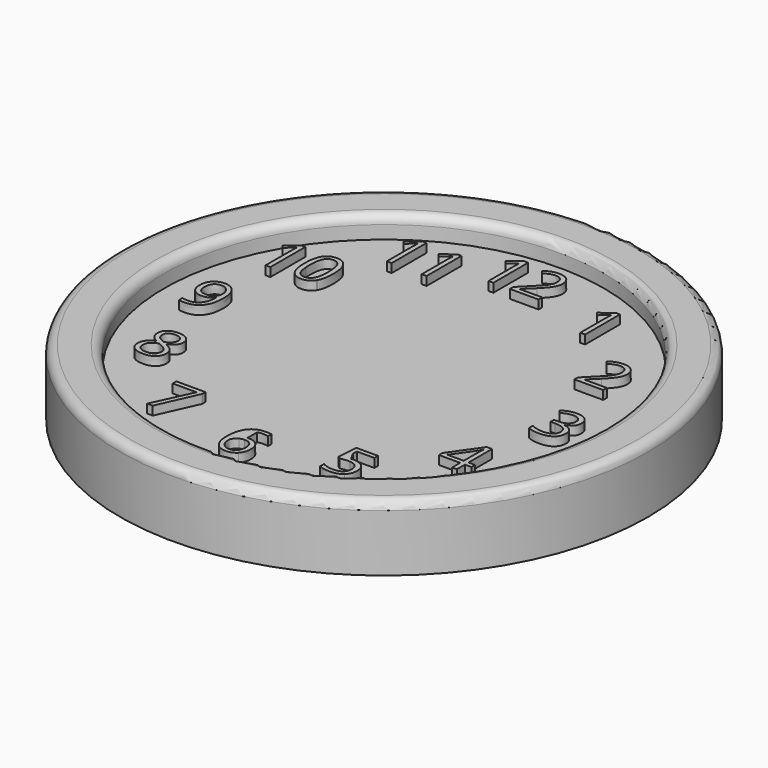
from build123d import *

# Parameters (mm, degrees)
F0_R         = 127
F1_DEPTH     = 25.4
F0_R_2       = 152.4
F2_DEPTH     = 38.1
F3_R         = 5.08
F5_TEXT_SIZE = 35.2777777778
F6_DEPTH     = 5.08


# Not quite as in the source:
# - Text() gives the source's letters only with a copy of the font that has no kerning and outlines rounded to 1/6400 em; it was checked with that copy


with BuildPart() as f1:
    # F0 (on Top) → F1 (new body)
    with BuildSketch(Plane.XY):
        Circle(F0_R)
    extrude(amount=F1_DEPTH)


with BuildPart() as f2:
    # F0 (on Top) → F2 (new body)
    with BuildSketch(Plane.XY):
        Circle(F0_R_2)
        Circle(F0_R, mode=Mode.SUBTRACT)
    extrude(amount=F2_DEPTH)

    # F3
    f3_edges = [f2.edges().sort_by_distance(p)[0] for p in [
        (-127, 0, 38.1),
        (-152.4, 0, 38.1),
    ]]
    fillet(f3_edges, radius=F3_R)


with BuildPart() as f6:
    # F5 (on offset) → F6 (new body)
    with BuildSketch(Plane.XY.offset(25.654)):
        with BuildLine():
            add(Edge.make_bspline(
                [(0, -89.0715853715), (1.4167514722, -88.7566840278), (3.0702690972, -88.7566840278)],
                knots=[0.7073397651, 0.7073397651, 0.7073397651, 1, 1, 1], degree=2))
            Line((0, -89.0715853715), (0, -91.5732459323))
            add(Edge.make_bspline(
                [(3.1033420139, -91.1158854167), (1.3779739805, -91.1158854167), (0, -91.5732459323)],
                knots=[0, 0, 0, 0.4258661898, 0.4258661898, 0.4258661898], degree=2))
            add(Edge.make_bspline(
                [(6.1350260417, -91.5458333333), (4.8065972222, -91.1158854167), (3.1033420139, -91.1158854167)],
                knots=[0, 0, 0, 1, 1, 1], degree=2))
            Line((6.1350260417, -91.5458333333), (6.1350260417, -89.0819010417))
            add(Edge.make_bspline(
                [(3.0702690972, -88.7566840278), (5.0160590278, -88.7566840278), (6.1350260417, -89.0819010417)],
                knots=[0, 0, 0, 1, 1, 1], degree=2))
        make_face()
        with BuildLine():
            Line((0, -91.5732459323), (0, -89.0715853715))
            add(Edge.make_bspline(
                [(-5.4652994792, -92.4332899306), (-3.4241913797, -89.832680375), (0, -89.0715853715)],
                knots=[0, 0, 0, 0.7073397651, 0.7073397651, 0.7073397651], degree=2))
            add(Edge.make_bspline(
                [(-8.3509114583, -103.534765625), (-8.3509114583, -96.1098958333), (-5.4652994792, -92.4332899306)],
                knots=[0, 0, 0, 1, 1, 1], degree=2))
            add(Edge.make_bspline(
                [(-6.0606119792, -111.7092881944), (-8.3509114583, -108.7713107639), (-8.3509114583, -103.534765625)],
                knots=[0, 0, 0, 1, 1, 1], degree=2))
            add(Edge.make_bspline(
                [(0.1378038194, -114.647265625), (-3.7703125, -114.647265625), (-6.0606119792, -111.7092881944)],
                knots=[0, 0, 0, 1, 1, 1], degree=2))
            add(Edge.make_bspline(
                [(5.9365885417, -112.3983072917), (3.7923611111, -114.647265625), (0.1378038194, -114.647265625)],
                knots=[0, 0, 0, 1, 1, 1], degree=2))
            add(Edge.make_bspline(
                [(8.0808159722, -106.2191840278), (8.0808159722, -110.1493489583), (5.9365885417, -112.3983072917)],
                knots=[0, 0, 0, 1, 1, 1], degree=2))
            add(Edge.make_bspline(
                [(6.1267578125, -100.657421875), (8.0808159722, -102.7079427083), (8.0808159722, -106.2191840278)],
                knots=[0, 0, 0, 1, 1, 1], degree=2))
            add(Edge.make_bspline(
                [(0.7772135417, -98.6069010417), (4.1726996528, -98.6069010417), (6.1267578125, -100.657421875)],
                knots=[0, 0, 0, 1, 1, 1], degree=2))
            add(Edge.make_bspline(
                [(0, -98.6349784999), (0.378169054, -98.6069010417), (0.7772135417, -98.6069010417)],
                knots=[0.9026967975, 0.9026967975, 0.9026967975, 1, 1, 1], degree=2))
            add(Edge.make_bspline(
                [(-5.2200086806, -101.5724392361), (-3.5083325655, -98.8954574051), (0, -98.6349784999)],
                knots=[0, 0, 0, 0.9026967975, 0.9026967975, 0.9026967975], degree=2))
            Line((-5.2200086806, -101.5724392361), (-5.4239583333, -101.5724392361))
            add(Edge.make_bspline(
                [(-3.0840494792, -93.6376953125), (-5.2200086806, -96.1595052083), (-5.4239583333, -101.5724392361)],
                knots=[0, 0, 0, 1, 1, 1], degree=2))
            add(Edge.make_bspline(
                [(0, -91.5732459323), (-1.8577230845, -92.1898389885), (-3.0840494792, -93.6376953125)],
                knots=[0.4258661898, 0.4258661898, 0.4258661898, 1, 1, 1], degree=2))
        make_face()
        with BuildLine():
            add(Edge.make_bspline(
                [(0, -100.8653424744), (-1.4082443896, -100.9117606324), (-2.5989800347, -101.50078125)],
                knots=[0.0788056591, 0.0788056591, 0.0788056591, 1, 1, 1], degree=2))
            add(Edge.make_bspline(
                [(0.2425347222, -100.8613715278), (0.1204714602, -100.8613715278), (0, -100.8653424744)],
                knots=[0, 0, 0, 0.0788056591, 0.0788056591, 0.0788056591], degree=2))
            add(Edge.make_bspline(
                [(3.9963107639, -102.2917751736), (2.7395399306, -100.8613715278), (0.2425347222, -100.8613715278)],
                knots=[0, 0, 0, 1, 1, 1], degree=2))
            add(Edge.make_bspline(
                [(5.2530815972, -106.2191840278), (5.2530815972, -103.7221788194), (3.9963107639, -102.2917751736)],
                knots=[0, 0, 0, 1, 1, 1], degree=2))
            add(Edge.make_bspline(
                [(3.9026041667, -110.6730034722), (5.2530815972, -109.1296006944), (5.2530815972, -106.2191840278)],
                knots=[0, 0, 0, 1, 1, 1], degree=2))
            add(Edge.make_bspline(
                [(0.1047309028, -112.21640625), (2.5521267361, -112.21640625), (3.9026041667, -110.6730034722)],
                knots=[0, 0, 0, 1, 1, 1], degree=2))
            add(Edge.make_bspline(
                [(-2.7808810764, -111.3206814236), (-1.5158420139, -112.21640625), (0.1047309028, -112.21640625)],
                knots=[0, 0, 0, 1, 1, 1], degree=2))
            add(Edge.make_bspline(
                [(-4.7349392361, -108.892578125), (-4.0459201389, -110.4249565972), (-2.7808810764, -111.3206814236)],
                knots=[0, 0, 0, 1, 1, 1], degree=2))
            add(Edge.make_bspline(
                [(-5.4239583333, -105.5852864583), (-5.4239583333, -107.3601996528), (-4.7349392361, -108.892578125)],
                knots=[0, 0, 0, 1, 1, 1], degree=2))
            add(Edge.make_bspline(
                [(-4.6577690972, -103.2591579861), (-5.4239583333, -104.378125), (-5.4239583333, -105.5852864583)],
                knots=[0, 0, 0, 1, 1, 1], degree=2))
            add(Edge.make_bspline(
                [(-2.5989800347, -101.50078125), (-3.8915798611, -102.1401909722), (-4.6577690972, -103.2591579861)],
                knots=[0, 0, 0, 1, 1, 1], degree=2))
        make_face(mode=Mode.SUBTRACT)
        Polygon((44.4279513889, -75.5031549828), (44.3256858106, -76.7743399042), (46.6502291754, -80.8005671165), (46.8753472222, -78.1379640106), (56.9515625, -78.1379640106), (56.9515625, -75.5031549828), align=None)
        with BuildLine():
            Line((46.6502291754, -80.8005671165), (44.3256858106, -76.7743399042))
            Line((44.3256858106, -76.7743399042), (43.4798611111, -87.2881376217))
            Line((43.4798611111, -87.2881376217), (44.9626302083, -88.2362278995))
            add(Edge.make_bspline(
                [(49.3392795139, -87.7346219967), (47.7021701389, -87.7346219967), (44.9626302083, -88.2362278995)],
                knots=[0, 0, 0, 1, 1, 1], degree=2))
            add(Edge.make_bspline(
                [(50.690992768, -87.7993749604), (50.0547939445, -87.7346219967), (49.3392795139, -87.7346219967)],
                knots=[0.8891488365, 0.8891488365, 0.8891488365, 1, 1, 1], degree=2))
            Line((50.690992768, -87.7993749604), (49.2626542608, -85.3254200954))
            add(Edge.make_bspline(
                [(46.2359375, -85.7006376217), (47.7525335288, -85.3964735157), (49.2626542608, -85.3254200954)],
                knots=[0, 0, 0, 0.7663977475, 0.7663977475, 0.7663977475], degree=2))
            Line((46.2359375, -85.7006376217), (46.6502291754, -80.8005671165))
        make_face()
        with BuildLine():
            add(Edge.make_bspline(
                [(-71.6590054686, 41.3723460972), (-71.7749145216, 41.167531428), (-71.8982070662, 40.9745876736)],
                knots=[0.9401140472, 0.9401140472, 0.9401140472, 1, 1, 1], degree=2))
            Line((-71.6590054686, 41.3723460972), (-74.0546251018, 42.7554577373))
            add(Edge.make_bspline(
                [(-78.1958416148, 40.2166666667), (-75.3363356992, 40.2166666667), (-74.0546251018, 42.7554577373)],
                knots=[0, 0, 0, 0.9995451018, 0.9995451018, 0.9995451018], degree=2))
            add(Edge.make_bspline(
                [(-82.3106636634, 42.7246961806), (-81.018063837, 40.2166666667), (-78.1958416148, 40.2166666667)],
                knots=[0, 0, 0, 1, 1, 1], degree=2))
            add(Edge.make_bspline(
                [(-83.5262787662, 48.2239195301), (-83.2878107352, 44.6206531855), (-82.3106636634, 42.7246961806)],
                knots=[0.2440451779, 0.2440451779, 0.2440451779, 1, 1, 1], degree=2))
            Line((-83.5262787662, 48.2239195301), (-86.4886726615, 49.934258443))
            add(Edge.make_bspline(
                [(-84.3777209551, 41.0517578125), (-86.3631522517, 44.1422145902), (-86.4886726615, 49.934258443)],
                knots=[0, 0, 0, 0.9367792731, 0.9367792731, 0.9367792731], degree=2))
            add(Edge.make_bspline(
                [(-78.1958416148, 37.752734375), (-82.258298212, 37.752734375), (-84.3777209551, 41.0517578125)],
                knots=[0, 0, 0, 1, 1, 1], degree=2))
            add(Edge.make_bspline(
                [(-71.8982070662, 40.9745876736), (-73.9569961287, 37.752734375), (-78.1958416148, 37.752734375)],
                knots=[0, 0, 0, 1, 1, 1], degree=2))
        make_face()
        with BuildLine():
            Line((-74.0546251018, 42.7554577373), (-71.6590054686, 41.3723460972))
            add(Edge.make_bspline(
                [(-69.8394180037, 50.7283420139), (-69.8394180037, 44.5876100894), (-71.6590054686, 41.3723460972)],
                knots=[0, 0, 0, 0.9401140472, 0.9401140472, 0.9401140472], degree=2))
            add(Edge.make_bspline(
                [(-71.9671089759, 60.3553168403), (-69.8394180037, 57.0287326389), (-69.8394180037, 50.7283420139)],
                knots=[0, 0, 0, 1, 1, 1], degree=2))
            add(Edge.make_bspline(
                [(-78.1958416148, 63.6819010417), (-74.0947999481, 63.6819010417), (-71.9671089759, 60.3553168403)],
                knots=[0, 0, 0, 1, 1, 1], degree=2))
            add(Edge.make_bspline(
                [(-84.4466228648, 60.4931206597), (-82.3961020314, 63.6819010417), (-78.1958416148, 63.6819010417)],
                knots=[0, 0, 0, 1, 1, 1], degree=2))
            add(Edge.make_bspline(
                [(-86.4971436981, 50.7283420139), (-86.4971436981, 57.3043402778), (-84.4466228648, 60.4931206597)],
                knots=[0, 0, 0, 1, 1, 1], degree=2))
            add(Edge.make_bspline(
                [(-86.4886726615, 49.934258443), (-86.4971436981, 50.3251479866), (-86.4971436981, 50.7283420139)],
                knots=[0.9367792731, 0.9367792731, 0.9367792731, 1, 1, 1], degree=2))
            Line((-86.4886726615, 49.934258443), (-83.5262787662, 48.2239195301))
            add(Edge.make_bspline(
                [(-83.6032634898, 50.7283420139), (-83.6032634898, 49.3871633515), (-83.5262787662, 48.2239195301)],
                knots=[0, 0, 0, 0.2440451779, 0.2440451779, 0.2440451779], degree=2))
            add(Edge.make_bspline(
                [(-82.3106636634, 58.7126953125), (-83.6032634898, 56.2239583333), (-83.6032634898, 50.7283420139)],
                knots=[0, 0, 0, 1, 1, 1], degree=2))
            add(Edge.make_bspline(
                [(-78.1958416148, 61.2014322917), (-81.018063837, 61.2014322917), (-82.3106636634, 58.7126953125)],
                knots=[0, 0, 0, 1, 1, 1], degree=2))
            add(Edge.make_bspline(
                [(-74.0534588023, 58.6768663194), (-75.3350343231, 61.2014322917), (-78.1958416148, 61.2014322917)],
                knots=[0, 0, 0, 1, 1, 1], degree=2))
            add(Edge.make_bspline(
                [(-72.7718832814, 50.7283420139), (-72.7718832814, 56.1523003472), (-74.0534588023, 58.6768663194)],
                knots=[0, 0, 0, 1, 1, 1], degree=2))
            add(Edge.make_bspline(
                [(-74.0534588023, 42.7577690972), (-72.7718832814, 45.2988715278), (-72.7718832814, 50.7283420139)],
                knots=[0, 0, 0, 1, 1, 1], degree=2))
            add(Edge.make_bspline(
                [(-74.0546251018, 42.7554577373), (-74.0540417887, 42.7566131543), (-74.0534588023, 42.7577690972)],
                knots=[0.9995451018, 0.9995451018, 0.9995451018, 1, 1, 1], degree=2))
        make_face()
        with Locations((77.1127035939, -63.5)):
            Text('4', F5_TEXT_SIZE, font='Open Sans', text_align=(TextAlign.LEFT, TextAlign.BOTTOM))
        with Locations((-111.8829210069, -12.7)):
            Text('9', F5_TEXT_SIZE, font='Open Sans', text_align=(TextAlign.LEFT, TextAlign.BOTTOM))
        with Locations((91.4052734375, -12.7)):
            Text('3', F5_TEXT_SIZE, font='Open Sans', text_align=(TextAlign.LEFT, TextAlign.BOTTOM))
        with Locations((-98.3041749481, -63.5)):
            Text('8', F5_TEXT_SIZE, font='Open Sans', text_align=(TextAlign.LEFT, TextAlign.BOTTOM))
        Polygon((-42.7550130208, -75.5031549828), (-43.591766854, -75.5031549828), (-48.5063558794, -84.0154728732), (-56.2212022569, -100.6881810245), (-53.0517144097, -100.6881810245), (-42.7550130208, -77.7962105384), align=None)
        Polygon((-48.5063558794, -84.0154728732), (-43.591766854, -75.5031549828), (-59.5119574653, -75.5031549828), (-59.5119574653, -78.1379640106), (-45.7866970486, -78.1379640106), align=None)
        with BuildLine():
            Line((0, -98.6349784999), (0, -91.5732459323))
            add(Edge.make_bspline(
                [(0, -91.5732459323), (-1.8577230845, -92.1898389885), (-3.0840494792, -93.6376953125)],
                knots=[0.4258661898, 0.4258661898, 0.4258661898, 1, 1, 1], degree=2))
            add(Edge.make_bspline(
                [(-3.0840494792, -93.6376953125), (-5.2200086806, -96.1595052083), (-5.4239583333, -101.5724392361)],
                knots=[0, 0, 0, 1, 1, 1], degree=2))
            Line((-5.4239583333, -101.5724392361), (-5.2200086806, -101.5724392361))
            add(Edge.make_bspline(
                [(-5.2200086806, -101.5724392361), (-3.5083325655, -98.8954574051), (0, -98.6349784999)],
                knots=[0, 0, 0, 0.9026967975, 0.9026967975, 0.9026967975], degree=2))
        make_face()
        with BuildLine():
            Line((49.2626542608, -85.3254200954), (46.6502291754, -80.8005671165))
            Line((46.6502291754, -80.8005671165), (46.2359375, -85.7006376217))
            add(Edge.make_bspline(
                [(46.2359375, -85.7006376217), (47.7525335288, -85.3964735157), (49.2626542608, -85.3254200954)],
                knots=[0, 0, 0, 0.7663977475, 0.7663977475, 0.7663977475], degree=2))
        make_face()
        with BuildLine():
            add(Edge.make_bspline(
                [(49.2626542608, -85.3254200954), (49.7229473731, -85.3037626217), (50.1826388889, -85.3037626217)],
                knots=[0.7663977475, 0.7663977475, 0.7663977475, 1, 1, 1], degree=2))
            Line((49.2626542608, -85.3254200954), (50.690992768, -87.7993749604))
            add(Edge.make_bspline(
                [(55.7940104167, -93.0042400523), (55.7940104167, -88.3187652894), (50.690992768, -87.7993749604)],
                knots=[0, 0, 0, 0.8891488365, 0.8891488365, 0.8891488365], degree=2))
            add(Edge.make_bspline(
                [(54.1155598958, -97.141110712), (55.7940104167, -95.7107070662), (55.7940104167, -93.0042400523)],
                knots=[0, 0, 0, 1, 1, 1], degree=2))
            add(Edge.make_bspline(
                [(49.4054253472, -98.5715143578), (52.437109375, -98.5715143578), (54.1155598958, -97.141110712)],
                knots=[0, 0, 0, 1, 1, 1], degree=2))
            add(Edge.make_bspline(
                [(45.8721354167, -98.1305421356), (47.6635850694, -98.5715143578), (49.4054253472, -98.5715143578)],
                knots=[0, 0, 0, 1, 1, 1], degree=2))
            add(Edge.make_bspline(
                [(42.8790364583, -96.9178685245), (44.0806857639, -97.6895699134), (45.8721354167, -98.1305421356)],
                knots=[0, 0, 0, 1, 1, 1], degree=2))
            Line((42.8790364583, -96.9178685245), (42.8790364583, -99.6739449134))
            add(Edge.make_bspline(
                [(49.3723524306, -101.0354466495), (45.1169704861, -101.0354466495), (42.8790364583, -99.6739449134)],
                knots=[0, 0, 0, 1, 1, 1], degree=2))
            add(Edge.make_bspline(
                [(56.2377387153, -98.8112930037), (53.7490017361, -101.0354466495), (49.3723524306, -101.0354466495)],
                knots=[0, 0, 0, 1, 1, 1], degree=2))
            add(Edge.make_bspline(
                [(58.7264756944, -92.6790230384), (58.7264756944, -96.5871393578), (56.2377387153, -98.8112930037)],
                knots=[0, 0, 0, 1, 1, 1], degree=2))
            add(Edge.make_bspline(
                [(56.4444444444, -87.2771133162), (58.7264756944, -89.2504640106), (58.7264756944, -92.6790230384)],
                knots=[0, 0, 0, 1, 1, 1], degree=2))
            add(Edge.make_bspline(
                [(50.1826388889, -85.3037626217), (54.1624131944, -85.3037626217), (56.4444444444, -87.2771133162)],
                knots=[0, 0, 0, 1, 1, 1], degree=2))
        make_face()
        with Locations((-20.3674045139, 88.9)):
            Text('12', F5_TEXT_SIZE, font='Open Sans', text_align=(TextAlign.LEFT, TextAlign.BOTTOM))
        with Locations((43.4991536458, 75.2881810245)):
            Text('1', F5_TEXT_SIZE, font='Open Sans', text_align=(TextAlign.LEFT, TextAlign.BOTTOM))
        with Locations((77.7052600176, 38.1)):
            Text('2', F5_TEXT_SIZE, font='Open Sans', text_align=(TextAlign.LEFT, TextAlign.BOTTOM))
        with BuildLine():
            Line((-98.8994874481, 38.1), (-96.1103381426, 38.1))
            Line((-96.1103381426, 38.1), (-96.1103381426, 63.2850260417))
            Line((-96.1103381426, 63.2850260417), (-98.5191489064, 63.2850260417))
            Line((-98.5191489064, 63.2850260417), (-105.1833416148, 58.1311631944))
            Line((-105.1833416148, 58.1311631944), (-103.6674996009, 56.1688368056))
            add(Edge.make_bspline(
                [(-99.5692140106, 59.5284939236), (-100.018454462, 59.134375), (-103.6674996009, 56.1688368056)],
                knots=[0, 0, 0, 1, 1, 1], degree=2))
            add(Edge.make_bspline(
                [(-98.7616836287, 60.2864149306), (-99.1199735592, 59.9226128472), (-99.5692140106, 59.5284939236)],
                knots=[0, 0, 0, 1, 1, 1], degree=2))
            add(Edge.make_bspline(
                [(-98.8994874481, 56.0475694444), (-98.8994874481, 58.291015625), (-98.7616836287, 60.2864149306)],
                knots=[0, 0, 0, 1, 1, 1], degree=2))
            Line((-98.8994874481, 56.0475694444), (-98.8994874481, 38.1))
        make_face()
        with Locations((-68.1853298611, 75.2881810245)):
            Text('11', F5_TEXT_SIZE, font='Open Sans', text_align=(TextAlign.LEFT, TextAlign.BOTTOM))
    extrude(amount=F6_DEPTH)


solid = Compound([f1.part, f2.part, f6.part])
